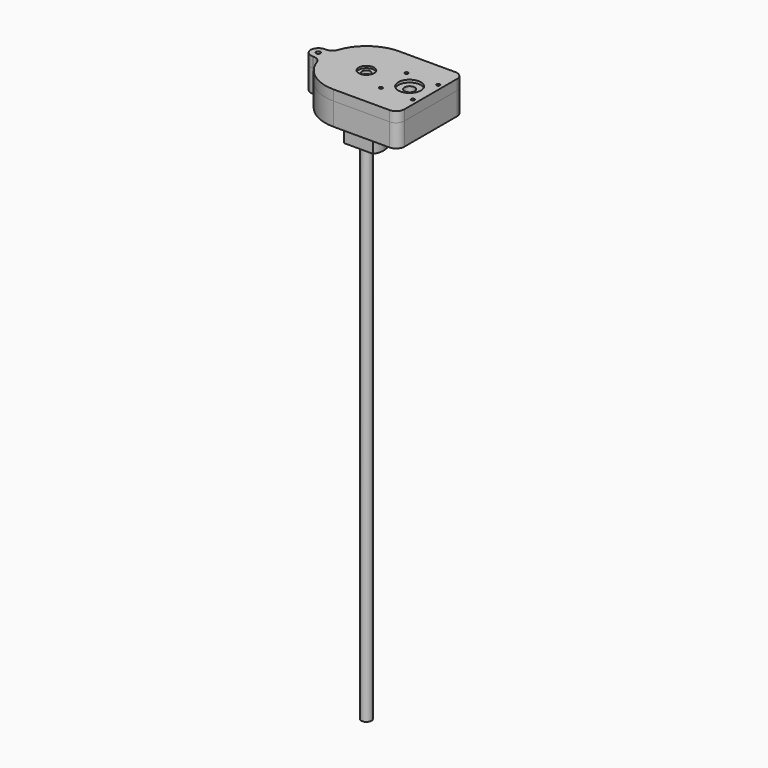
from build123d import *

# Parameters (mm, degrees)
F0_R           = 17
F0_R_2         = 3.75
F0_R_3         = 5
F1_DEPTH       = 8
F2_DEPTH       = 25
F3_DEPTH       = 15
F4_R           = 4
F5_DEPTH       = 10
F6_R           = 3
F7_DEPTH       = 30
F8_R           = 3.5
F8_R_2         = 2.1
F9_DEPTH       = 29
F8_R_3         = 17
F8_R_4         = 3.75
F8_R_5         = 5.5
F10_DEPTH      = 4
F11_R          = 2.1
F11_R_2        = 3.75
F11_R_3        = 5.5
F12_DEPTH      = 4
F13_R          = 5
F14_DEPTH      = 6
F15_R          = 3
F16_DEPTH      = 25
F15_R_2        = 1.6
F17_DEPTH      = 12
F15_W          = 22.5
F15_H          = 80
F18_DEPTH      = 25
F19_R          = 2.1
F20_DEPTH      = 12
F21_R          = 1.6
F21_R_2        = 2.1
F21_R_3        = 11
F21_R_4        = 5
F22_DEPTH      = 10
F23_R          = 2.1
F23_R_2        = 17
F23_R_3        = 3
F24_DEPTH      = 2
F25_R          = 11
F25_R_2        = 4
F26_DEPTH      = 4
F27_DEPTH      = 3
F28_R          = 11
F29_DEPTH      = 8
F30_R          = 1.6
F31_DEPTH      = 3
F32_DEPTH      = 25
F33_R          = 1.6
F34_DEPTH      = 3
F35_R          = 2.1
F36_DEPTH      = 4
F37_T1_DEPTH   = 22
F37_T3_DEPTH   = 12
F37_T5_DEPTH   = 62
F37_2_T1_DEPTH = 10
F37_2_T3_DEPTH = 50
F38_R          = 7.5
F39_DEPTH      = 25
F40_R          = 11
F40_R_2        = 5
F41_DEPTH      = 2.5
F42_R          = 3.75
F42_R_2        = 5
F43_DEPTH      = 25
F44_R          = 3.75
F44_R_2        = 1.6
F45_DEPTH      = 4
F46_DEPTH      = 500


# Not quite as in the source:
# - a fillet or chamfer that OpenCascade refuses, or shapes differently, is made with other operations: its cross-section is extruded or revolved along the edge and cut away or added
# - a feature names something its author has since deleted; it is built from what else it names


with BuildPart() as f1:
    # F0 (on Top) → F1 (new body)
    with BuildSketch(Plane.XY):
        Circle(F0_R)
        with Locations((-11, 0)):
            Circle(F0_R_2, mode=Mode.SUBTRACT)
        Circle(F0_R_3, mode=Mode.SUBTRACT)
        with Locations((11, 0)):
            Circle(F0_R_2, mode=Mode.SUBTRACT)
    extrude(amount=-F1_DEPTH)


with BuildPart() as f2:
    # F0 (on Top) → F2 (new body)
    with BuildSketch(Plane.XY):
        Circle(F0_R_3)
    extrude(amount=-F2_DEPTH)

    # F3 (add): a face of the model
    f3_faces = [f2.faces().sort_by_distance(p)[0] for p in [
        (0, 0, 0),
    ]]
    extrude(f3_faces, amount=F3_DEPTH)

    # F4 (on face) → F5 (join)
    with BuildSketch(Plane.XY.offset(15)):
        Circle(F4_R)
    extrude(amount=F5_DEPTH)

    # F6 (on face) → F7 (cut)
    with BuildSketch(Plane.XY.offset(25)):
        Circle(F6_R)
    extrude(amount=-F7_DEPTH, mode=Mode.SUBTRACT)

    # F46 (add): a face of the model
    f46_faces = [f2.faces().sort_by_distance(p)[0] for p in [
        (0, 0, -25),
    ]]
    extrude(f46_faces, amount=F46_DEPTH)


with BuildPart() as f9:
    # F8 (on face) → F9 (new body)
    with BuildSketch(Plane.XY):
        with Locations((-11, 0)):
            Circle(F8_R)
        with Locations((-11, 0)):
            Circle(F8_R_2, mode=Mode.SUBTRACT)
    extrude(amount=-F9_DEPTH)


with BuildPart() as f9b:
    # F8 (on face) → F9, piece 2 (new body)
    with BuildSketch(Plane.XY):
        with Locations((11, 0)):
            Circle(F8_R)
        with Locations((11, 0)):
            Circle(F8_R_2, mode=Mode.SUBTRACT)
    extrude(amount=-F9_DEPTH)


with BuildPart() as f10:
    # F8 (on face) → F10 (new body)
    with BuildSketch(Plane.XY):
        with BuildLine():
            Line((85, 40), (0, 40))
            ThreePointArc((0, 40), (-25.495097568, 30.8220700148), (-39.2905841138, 7.5))
            ThreePointArc((-39.2905841138, 7.5), (-40, 0), (-39.2905841138, -7.5))
            ThreePointArc((-39.2905841138, -7.5), (-25.495097568, -30.8220700148), (0, -40))
            Line((0, -40), (85, -40))
            Line((85, -40), (85, 40))
        make_face()
        Circle(F8_R_3, mode=Mode.SUBTRACT)
        Circle(F8_R_3)
        with Locations((-11, 0)):
            Circle(F8_R_4, mode=Mode.SUBTRACT)
        Circle(F8_R_5, mode=Mode.SUBTRACT)
        with Locations((11, 0)):
            Circle(F8_R_4, mode=Mode.SUBTRACT)
        with Locations((-11, 0)):
            Circle(F8_R_4)
        with Locations((-11, 0)):
            Circle(F8_R, mode=Mode.SUBTRACT)
        with Locations((-11, 0)):
            Circle(F8_R)
        with Locations((-11, 0)):
            Circle(F8_R_2, mode=Mode.SUBTRACT)
        with Locations((11, 0)):
            Circle(F8_R_4)
        with Locations((11, 0)):
            Circle(F8_R, mode=Mode.SUBTRACT)
        with Locations((11, 0)):
            Circle(F8_R)
        with Locations((11, 0)):
            Circle(F8_R_2, mode=Mode.SUBTRACT)
        with BuildLine():
            ThreePointArc((-39.2905841138, -7.5), (-40, 0), (-39.2905841138, 7.5))
            Line((-39.2905841138, 7.5), (-54.2905841138, 7.5))
            Line((-54.2905841138, 7.5), (-54.2905841138, -7.5))
            Line((-54.2905841138, -7.5), (-39.2905841138, -7.5))
        make_face()
        with Locations((-46.7905841138, 0)):
            Circle(F8_R_2, mode=Mode.SUBTRACT)
    extrude(amount=F10_DEPTH)

    # F11 (on face) → F12 (join)
    with BuildSketch(Plane.XY.offset(4)):
        with BuildLine():
            ThreePointArc((-39.2905841138, -7.5), (-25.495097568, -30.8220700148), (0, -40))
            Line((0, -40), (85, -40))
            Line((85, -40), (85, 40))
            Line((85, 40), (0, 40))
            ThreePointArc((0, 40), (-25.495097568, 30.8220700148), (-39.2905841138, 7.5))
            Line((-39.2905841138, 7.5), (-54.2905841138, 7.5))
            Line((-54.2905841138, 7.5), (-54.2905841138, -7.5))
            Line((-54.2905841138, -7.5), (-39.2905841138, -7.5))
        make_face()
        with Locations((-46.7905841138, 0)):
            Circle(F11_R, mode=Mode.SUBTRACT)
        with Locations((-11, 0)):
            Circle(F11_R_2, mode=Mode.SUBTRACT)
        Circle(F11_R_3, mode=Mode.SUBTRACT)
        with Locations((11, 0)):
            Circle(F11_R_2, mode=Mode.SUBTRACT)
    extrude(amount=F12_DEPTH)

    # F15 (on face) → F16 (cut)
    with BuildSketch(Plane.XY.offset(8)):
        with Locations((42, 0)):
            Circle(F15_R)
    extrude(amount=-F16_DEPTH, mode=Mode.SUBTRACT)

    # F15 (on face) → F17 (join)
    with BuildSketch(Plane.XY.offset(8)):
        with BuildLine():
            Line((62.5, 40), (52.5, 40))
            Line((52.5, 40), (52.5, 7.6648548584))
            ThreePointArc((52.5, 7.6648548584), (54.3592070943, 4.0311288741), (55, 0))
            ThreePointArc((55, 0), (54.3592070943, -4.0311288741), (52.5, -7.6648548584))
            Line((52.5, -7.6648548584), (52.5, -40))
            Line((52.5, -40), (62.5, -40))
            Line((62.5, -40), (62.5, 40))
        make_face()
        with Locations((57.5, -15.5)):
            Circle(F15_R_2, mode=Mode.SUBTRACT)
        with Locations((57.5, 15.5)):
            Circle(F15_R_2, mode=Mode.SUBTRACT)
    extrude(amount=F17_DEPTH)

    # F15 (on face) → F18 (cut)
    with BuildSketch(Plane.XY.offset(8)):
        with Locations((73.75, 0)):
            Rectangle(F15_W, F15_H)
    extrude(amount=-F18_DEPTH, mode=Mode.SUBTRACT)

    # F19 (on face) → F20 (join, through all)
    with BuildSketch(Plane.XY.offset(8)):
        with BuildLine():
            ThreePointArc((0, -37), (-37, 0), (0, 37))
            Line((0, 37), (52.5, 37))
            Line((52.5, 37), (52.5, 40))
            Line((52.5, 40), (0, 40))
            ThreePointArc((0, 40), (-25.495097568, 30.8220700148), (-39.2905841138, 7.5))
            Line((-39.2905841138, 7.5), (-54.2905841138, 7.5))
            Line((-54.2905841138, 7.5), (-54.2905841138, -7.5))
            Line((-54.2905841138, -7.5), (-39.2905841138, -7.5))
            ThreePointArc((-39.2905841138, -7.5), (-25.495097568, -30.8220700148), (0, -40))
            Line((0, -40), (52.5, -40))
            Line((52.5, -40), (52.5, -37))
            Line((52.5, -37), (0, -37))
        make_face()
        with Locations((-46.7905841138, 0)):
            Circle(F19_R, mode=Mode.SUBTRACT)
    extrude(amount=F20_DEPTH)

    # F23 (on face) → F24 (join)
    with BuildSketch(Plane(origin=(0, 0, 0), x_dir=(1, 0, 0), z_dir=(0, 0, -1))):
        with BuildLine():
            Line((62.5, 40), (0, 40))
            ThreePointArc((0, 40), (-25.495097568, 30.8220700148), (-39.2905841138, 7.5))
            Line((-39.2905841138, 7.5), (-54.2905841138, 7.5))
            Line((-54.2905841138, 7.5), (-54.2905841138, -7.5))
            Line((-54.2905841138, -7.5), (-39.2905841138, -7.5))
            ThreePointArc((-39.2905841138, -7.5), (-25.495097568, -30.8220700148), (0, -40))
            Line((0, -40), (62.5, -40))
            Line((62.5, -40), (62.5, 40))
        make_face()
        with Locations((-46.7905841138, 0)):
            Circle(F23_R, mode=Mode.SUBTRACT)
        Circle(F23_R_2, mode=Mode.SUBTRACT)
        with Locations((42, 0)):
            Circle(F23_R_3, mode=Mode.SUBTRACT)
    extrude(amount=F24_DEPTH)

    # F32 (cut): faces of the model
    f32_faces = [f10.faces().sort_by_distance(p)[0] for p in [
        (57.5, 15.5, 8),
        (57.5, -15.5, 8),
    ]]
    extrude(f32_faces, amount=-F32_DEPTH, mode=Mode.SUBTRACT)

    # F33 (on face) → F34 (cut)
    with BuildSketch(Plane(origin=(0, 0, -2), x_dir=(1, 0, 0), z_dir=(0, 0, -1))):
        Polygon((54.7, -13.8834192463), (54.7, -17.1165807537), (57.5, -18.7331615075), (60.3, -17.1165807537), (60.3, -13.8834192463), (57.5, -12.2668384925), align=None)
        with Locations((57.5, -15.5)):
            Circle(F33_R, mode=Mode.SUBTRACT)
        Polygon((54.7, 17.1165807537), (54.7, 13.8834192463), (57.5, 12.2668384925), (60.3, 13.8834192463), (60.3, 17.1165807537), (57.5, 18.7331615075), align=None)
        with Locations((57.5, 15.5)):
            Circle(F33_R, mode=Mode.SUBTRACT)
    extrude(amount=-F34_DEPTH, mode=Mode.SUBTRACT)

    # F35 (on face) → F36 (cut)
    with BuildSketch(Plane(origin=(0, 0, -2), x_dir=(1, 0, 0), z_dir=(0, 0, -1))):
        Polygon((-50.2905841138, 2.0207259422), (-50.2905841138, -2.0207259422), (-46.7905841138, -4.0414518843), (-43.2905841138, -2.0207259422), (-43.2905841138, 2.0207259422), (-46.7905841138, 4.0414518843), align=None)
        with Locations((-46.7905841138, 0)):
            Circle(F35_R, mode=Mode.SUBTRACT)
    extrude(amount=-F36_DEPTH, mode=Mode.SUBTRACT)

    # F37: fillet of radius 8 on 8 edges, made by hand

    # F37_s2 → F37_t1 (join)
    with BuildSketch(Plane.XY.offset(-2)):
        with BuildLine():
            ThreePointArc((-37.8570960617, -12.9166666667), (-40.7737685927, -8.9935929014), (-45.428515274, -7.5))
            Line((-45.428515274, -7.5), (-39.2905841138, -7.5))
            ThreePointArc((-39.2905841138, -7.5), (-38.6688014885, -10.2334642934), (-37.8570960617, -12.9166666667))
        make_face()
        with BuildLine():
            ThreePointArc((-37.8570960617, 12.9166666667), (-40.7737685927, 8.9935929014), (-45.428515274, 7.5))
            Line((-45.428515274, 7.5), (-39.2905841138, 7.5))
            ThreePointArc((-39.2905841138, 7.5), (-38.6688014885, 10.2334642934), (-37.8570960617, 12.9166666667))
        make_face()
    extrude(amount=F37_T1_DEPTH)

    # F37_s4 → F37_t3 (join)
    with BuildSketch(Plane.XY.offset(8)):
        with BuildLine():
            ThreePointArc((52.5, 29), (50.1568542495, 34.6568542495), (44.5, 37))
            Line((44.5, 37), (52.5, 37))
            Line((52.5, 37), (52.5, 29))
        make_face()
        with BuildLine():
            ThreePointArc((52.5, -29), (50.1568542495, -34.6568542495), (44.5, -37))
            Line((44.5, -37), (52.5, -37))
            Line((52.5, -37), (52.5, -29))
        make_face()
    extrude(amount=F37_T3_DEPTH)

    # F37_s6 → F37_t5 (cut)
    with BuildSketch(Plane.XY.offset(-22)):
        with BuildLine():
            ThreePointArc((-54.2905841138, 0.5), (-51.9474383632, -5.1568542495), (-46.2905841138, -7.5))
            Line((-46.2905841138, -7.5), (-54.2905841138, -7.5))
            Line((-54.2905841138, -7.5), (-54.2905841138, 0.5))
        make_face()
        with BuildLine():
            ThreePointArc((-46.2905841138, 7.5), (-51.9474383632, 5.1568542495), (-54.2905841138, -0.5))
            Line((-54.2905841138, -0.5), (-54.2905841138, 7.5))
            Line((-54.2905841138, 7.5), (-46.2905841138, 7.5))
        make_face()
        with BuildLine():
            ThreePointArc((54.5, -40), (60.1568542495, -37.6568542495), (62.5, -32))
            Line((62.5, -32), (62.5, -40))
            Line((62.5, -40), (54.5, -40))
        make_face()
        with BuildLine():
            ThreePointArc((62.5, 32), (60.1568542495, 37.6568542495), (54.5, 40))
            Line((54.5, 40), (62.5, 40))
            Line((62.5, 40), (62.5, 32))
        make_face()
    extrude(amount=F37_T5_DEPTH, mode=Mode.SUBTRACT)


with BuildPart() as f14:
    # F13 (on face) → F14 (new body)
    with BuildSketch(Plane.XY.offset(15)):
        Polygon((4.9074772881, 8.5), (-4.9074772881, 8.5), (-9.8149545762, 0), (-4.9074772881, -8.5), (4.9074772881, -8.5), (9.8149545762, 0), align=None)
        Circle(F13_R, mode=Mode.SUBTRACT)
    extrude(amount=-F14_DEPTH)


with BuildPart() as f22:
    # F21 (on face) → F22 (new body)
    with BuildSketch(Plane.XY.offset(20)):
        with BuildLine():
            Line((0, -40), (62.5, -40))
            Line((62.5, -40), (62.5, 40))
            Line((62.5, 40), (0, 40))
            ThreePointArc((0, 40), (-25.495097568, 30.8220700148), (-39.2905841138, 7.5))
            Line((-39.2905841138, 7.5), (-54.2905841138, 7.5))
            Line((-54.2905841138, 7.5), (-54.2905841138, -7.5))
            Line((-54.2905841138, -7.5), (-39.2905841138, -7.5))
            ThreePointArc((-39.2905841138, -7.5), (-25.495097568, -30.8220700148), (0, -40))
        make_face()
        with Locations((57.5, -15.5)):
            Circle(F21_R, mode=Mode.SUBTRACT)
        with Locations((-46.7905841138, 0)):
            Circle(F21_R_2, mode=Mode.SUBTRACT)
        with BuildLine():
            Line((0, 37), (52.5, 37))
            Line((52.5, 37), (52.5, 7.6648548584))
            ThreePointArc((52.5, 7.6648548584), (55, 0), (52.5, -7.6648548584))
            Line((52.5, -7.6648548584), (52.5, -37))
            Line((52.5, -37), (0, -37))
            ThreePointArc((0, -37), (-37, 0), (0, 37))
        make_face(mode=Mode.SUBTRACT)
        with Locations((57.5, 15.5)):
            Circle(F21_R, mode=Mode.SUBTRACT)
        with BuildLine():
            Line((52.5, 7.6648548584), (52.5, 37))
            Line((52.5, 37), (0, 37))
            ThreePointArc((0, 37), (-37, 0), (0, -37))
            Line((0, -37), (52.5, -37))
            Line((52.5, -37), (52.5, -7.6648548584))
            ThreePointArc((52.5, -7.6648548584), (55, 0), (52.5, 7.6648548584))
        make_face()
        with Locations((26.5, -15.5)):
            Circle(F21_R, mode=Mode.SUBTRACT)
        with Locations((26.5, 15.5)):
            Circle(F21_R, mode=Mode.SUBTRACT)
        with Locations((42, 0)):
            Circle(F21_R_3, mode=Mode.SUBTRACT)
        with Locations((42, 0)):
            Circle(F21_R_3)
        with Locations((42, 0)):
            Circle(F21_R_4, mode=Mode.SUBTRACT)
    extrude(amount=F22_DEPTH)

    # F28 (on face) → F29 (cut)
    with BuildSketch(Plane(origin=(0, 0, 20), x_dir=(1, 0, 0), z_dir=(0, 0, -1))):
        Circle(F28_R)
    extrude(amount=-F29_DEPTH, mode=Mode.SUBTRACT)

    # F30 (on face) → F31 (cut)
    with BuildSketch(Plane(origin=(0, 0, 20), x_dir=(1, 0, 0), z_dir=(0, 0, -1))):
        Polygon((29.3, 13.8834192463), (29.3, 17.1165807537), (26.5, 18.7331615075), (23.7, 17.1165807537), (23.7, 13.8834192463), (26.5, 12.2668384925), align=None)
        with Locations((26.5, 15.5)):
            Circle(F30_R, mode=Mode.SUBTRACT)
        Polygon((29.3, -17.1165807537), (29.3, -13.8834192463), (26.5, -12.2668384925), (23.7, -13.8834192463), (23.7, -17.1165807537), (26.5, -18.7331615075), align=None)
        with Locations((26.5, -15.5)):
            Circle(F30_R, mode=Mode.SUBTRACT)
    extrude(amount=-F31_DEPTH, mode=Mode.SUBTRACT)

    # F37#2: fillet of radius 8 on 6 edges, made by hand

    # F37_2_s2 → F37_2_t1 (join)
    with BuildSketch(Plane.XY.offset(20)):
        with BuildLine():
            ThreePointArc((-45.428515274, -7.5), (-40.7737685927, -8.9935929014), (-37.8570960617, -12.9166666667))
            ThreePointArc((-37.8570960617, -12.9166666667), (-38.6688014885, -10.2334642934), (-39.2905841138, -7.5))
            Line((-39.2905841138, -7.5), (-45.428515274, -7.5))
        make_face()
        with BuildLine():
            ThreePointArc((-45.428515274, 7.5), (-40.7737685927, 8.9935929014), (-37.8570960617, 12.9166666667))
            ThreePointArc((-37.8570960617, 12.9166666667), (-38.6688014885, 10.2334642934), (-39.2905841138, 7.5))
            Line((-39.2905841138, 7.5), (-45.428515274, 7.5))
        make_face()
    extrude(amount=F37_2_T1_DEPTH)

    # F37_2_s4 → F37_2_t3 (cut)
    with BuildSketch(Plane.XY):
        with BuildLine():
            ThreePointArc((62.5, -32), (60.1568542495, -37.6568542495), (54.5, -40))
            Line((54.5, -40), (62.5, -40))
            Line((62.5, -40), (62.5, -32))
        make_face()
        with BuildLine():
            ThreePointArc((54.5, 40), (60.1568542495, 37.6568542495), (62.5, 32))
            Line((62.5, 32), (62.5, 40))
            Line((62.5, 40), (54.5, 40))
        make_face()
        with BuildLine():
            ThreePointArc((-54.2905841138, 0.5), (-51.9474383632, -5.1568542495), (-46.2905841138, -7.5))
            Line((-46.2905841138, -7.5), (-54.2905841138, -7.5))
            Line((-54.2905841138, -7.5), (-54.2905841138, 0.5))
        make_face()
        with BuildLine():
            ThreePointArc((-46.2905841138, 7.5), (-51.9474383632, 5.1568542495), (-54.2905841138, -0.5))
            Line((-54.2905841138, -0.5), (-54.2905841138, 7.5))
            Line((-54.2905841138, 7.5), (-46.2905841138, 7.5))
        make_face()
    extrude(amount=F37_2_T3_DEPTH, mode=Mode.SUBTRACT)

    # F38 (on face) → F39 (cut)
    with BuildSketch(Plane(origin=(0, 0, 28), x_dir=(1, 0, 0), z_dir=(0, 0, -1))):
        Circle(F38_R)
    extrude(amount=-F39_DEPTH, mode=Mode.SUBTRACT)

    # F40 (on face) → F41 (cut)
    with BuildSketch(Plane.XY.offset(30)):
        with Locations((42, 0)):
            Circle(F40_R)
        with Locations((42, 0)):
            Circle(F40_R_2, mode=Mode.SUBTRACT)
    extrude(amount=-F41_DEPTH, mode=Mode.SUBTRACT)


with BuildPart() as f26:
    # F25 (on face) → F26 (new body)
    with BuildSketch(Plane.XY.offset(25)):
        Circle(F25_R)
        Circle(F25_R_2, mode=Mode.SUBTRACT)
    extrude(amount=-F26_DEPTH)

    # F27 (add): a face of the model
    f27_faces = [f26.faces().sort_by_distance(p)[0] for p in [
        (-10.6888730163, 0, 25),
    ]]
    extrude(f27_faces, amount=F27_DEPTH)


with BuildPart() as f43:
    # F42 (on face) → F43 (new body)
    with BuildSketch(Plane(origin=(0, 0, -8), x_dir=(1, 0, 0), z_dir=(0, 0, -1))):
        with BuildLine():
            Line((14.0978721799, 9.5), (-14.0978721799, 9.5))
            ThreePointArc((-14.0978721799, 9.5), (-17, 0), (-14.0978721799, -9.5))
            Line((-14.0978721799, -9.5), (14.0978721799, -9.5))
            ThreePointArc((14.0978721799, -9.5), (16.2582875337, -4.9666977431), (17, 0))
            ThreePointArc((17, 0), (16.2582875337, 4.9666977431), (14.0978721799, 9.5))
        make_face()
        with Locations((-11, 0)):
            Circle(F42_R, mode=Mode.SUBTRACT)
        Circle(F42_R_2, mode=Mode.SUBTRACT)
        with Locations((11, 0)):
            Circle(F42_R, mode=Mode.SUBTRACT)
    extrude(amount=F43_DEPTH)

    # F44 (on face) → F45 (join, through all)
    with BuildSketch(Plane(origin=(0, 0, -33), x_dir=(1, 0, 0), z_dir=(0, 0, -1))):
        with Locations((-11, 0)):
            Circle(F44_R)
        with Locations((-11, 0)):
            Circle(F44_R_2, mode=Mode.SUBTRACT)
        with Locations((11, 0)):
            Circle(F44_R)
        with Locations((11, 0)):
            Circle(F44_R_2, mode=Mode.SUBTRACT)
    extrude(amount=-F45_DEPTH)


solid = Compound([f1.part, f2.part, f9.part, f9b.part, f10.part, f14.part, f22.part, f26.part, f43.part])
